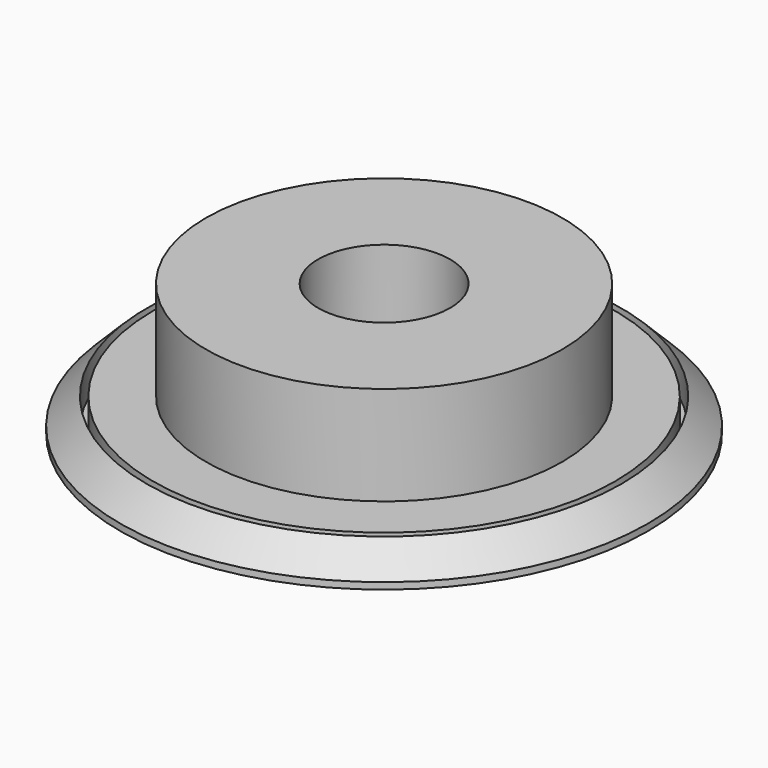
from build123d import *

# Parameters (mm, degrees)
F0_R     = 35
F0_R_2   = 10
F1_DEPTH = 5
F2_R     = 27
F2_R_2   = 10
F3_DEPTH = 15
F0_R_3   = 40
F4_DEPTH = 0.4
F5_R     = 40
F5_R_2   = 36
F6_DEPTH = 4.6
F7_SIZE  = 3.99999


# Not quite as in the source:
# - a fillet or chamfer is up to 0.001 mm smaller than in the source, because OpenCascade refuses the exact size


with BuildPart() as f1:
    # F0 (on Top) → F1 (new body)
    with BuildSketch(Plane.XY):
        Circle(F0_R)
        Circle(F0_R_2, mode=Mode.SUBTRACT)
    extrude(amount=F1_DEPTH)

    # F2 (on face) → F3 (join)
    with BuildSketch(Plane.XY.offset(5)):
        Circle(F2_R)
        Circle(F2_R_2, mode=Mode.SUBTRACT)
    extrude(amount=F3_DEPTH)

    # F0 (on Top) → F4 (join)
    with BuildSketch(Plane.XY):
        Circle(F0_R_3)
        Circle(F0_R, mode=Mode.SUBTRACT)
    extrude(amount=F4_DEPTH)

    # F5 (on face) → F6 (join)
    with BuildSketch(Plane.XY.offset(0.4)):
        Circle(F5_R)
        Circle(F5_R_2, mode=Mode.SUBTRACT)
    extrude(amount=F6_DEPTH)

    # F7 (size 4 in the source; OpenCascade refuses exactly that, so slightly less here)
    f7_edges = [f1.edges().sort_by_distance(p)[0] for p in [
        (-40, 0, 5),
    ]]
    chamfer(f7_edges, length=F7_SIZE)


solid = f1.part
